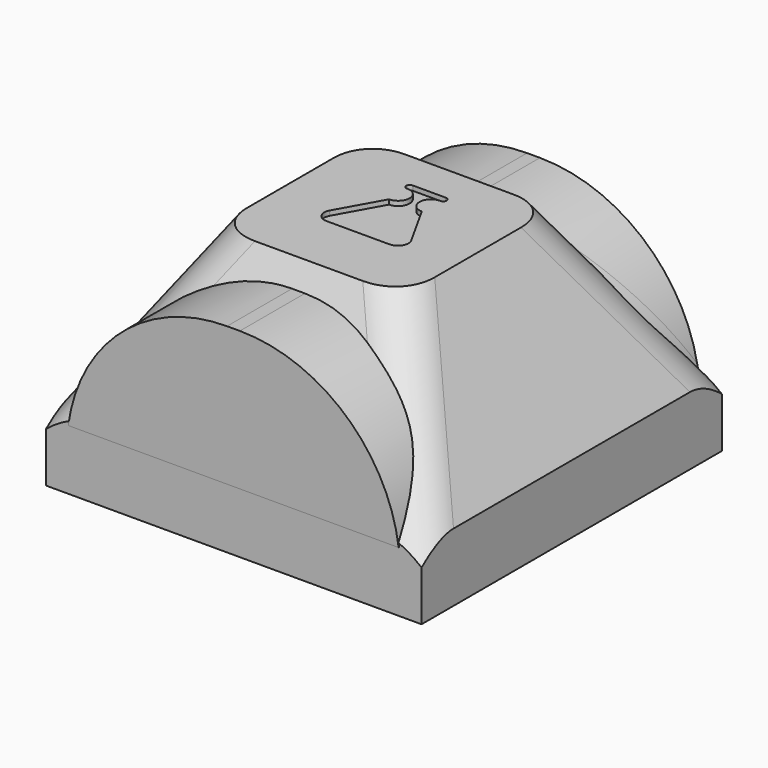
from build123d import *

# Parameters (mm, degrees)
F0_W          = 40.64
F0_H          = 40.64
F1_DEPTH      = 23.876
F2_SIZE2      = 10.16
F2_SIZE       = 16.51
F4_DEPTH      = 5.5372
F4_DEPTH_BACK = 35.052
F6_DEPTH      = 0.508
F7_T4_DEPTH   = 41.0469310155
F7_S5_R       = 17.3367265746
F7_T6_DEPTH   = 25
F7_T10_DEPTH  = 41.0469310155
F7_S11_R      = 17.3367265746
F7_T12_DEPTH  = 25
F7_T16_DEPTH  = 41.0469310155
F7_S17_R      = 17.3367265746
F7_T18_DEPTH  = 25
F7_T23_DEPTH  = 41.0469310155
F7_S24_R      = 17.3367265746
F7_T25_DEPTH  = 25
F7_T30_DEPTH  = 41.0469310155
F7_S31_R      = 17.3367265746
F7_T32_DEPTH  = 25
F7_T37_DEPTH  = 41.0469310155
F7_S39_R      = 17.3367265746
F7_T40_DEPTH  = 25
F7_T44_DEPTH  = 41.0469310155
F7_S46_R      = 17.3367265746
F7_T47_DEPTH  = 25
F7_T51_DEPTH  = 41.0469310155
F7_S53_R      = 17.3367265746
F7_T54_DEPTH  = 25


# Not quite as in the source:
# - a fillet or chamfer that OpenCascade refuses, or shapes differently, is made with other operations: its cross-section is extruded or revolved along the edge and cut away or added


with BuildPart() as f1:
    # F0 (on Top) → F1 (new body)
    with BuildSketch(Plane.XY):
        with Locations((-20.32, 14.8309261845)):
            Rectangle(F0_W, F0_H)
    extrude(amount=F1_DEPTH)

    # F2
    f2_edges = [f1.edges().sort_by_distance(p)[0] for p in [
        (0, 14.830926, 23.876),
        (-20.32, 35.150926, 23.876),
        (-40.64, 14.830926, 23.876),
        (-20.32, -5.489074, 23.876),
    ]]
    chamfer(f2_edges, length=F2_SIZE, length2=F2_SIZE2)

    # F3 (on Front) → F4 (join, two sides)
    with BuildSketch(Plane.XZ) as f4_sk:
        with BuildLine():
            Line((-19.622727835, 21.5899987397), (-21.017272165, 21.5899987397))
            ThreePointArc((-21.017272165, 21.5899987397), (-32.4394065874, 17.2953936781), (-38.2026230943, 6.5392734254))
            Line((-38.2026230943, 6.5392734254), (-2.4373769057, 6.5392734254))
            ThreePointArc((-2.4373769057, 6.5392734254), (-8.2005934126, 17.2953936781), (-19.622727835, 21.5899987397))
        make_face()
    extrude(amount=F4_DEPTH)
    extrude(f4_sk.sketch, amount=-F4_DEPTH_BACK)

    # F5 (on face) → F6 (cut)
    with BuildSketch(Plane.XY.offset(23.876)):
        with BuildLine():
            Line((-20.32, 11.3146617191), (-20.32, 20.958676386))
            Line((-20.32, 20.958676386), (-22.098, 20.958676386))
            ThreePointArc((-22.098, 20.958676386), (-22.5080143202, 20.5929218839), (-22.1218966733, 20.2020238648))
            ThreePointArc((-22.1218966733, 20.2020238648), (-20.8577108363, 18.9738562556), (-22.098, 17.7215606446))
            Line((-22.098, 17.7215606446), (-24.7307707736, 12.9957624854))
            ThreePointArc((-24.7307707736, 12.9957624854), (-24.7178678661, 11.8725673854), (-23.7429447999, 11.3146617191))
            Line((-23.7429447999, 11.3146617191), (-20.32, 11.3146617191))
        make_face()
        with BuildLine():
            Line((-18.542, 20.958676386), (-20.32, 20.958676386))
            Line((-20.32, 20.958676386), (-20.32, 11.3146617191))
            Line((-20.32, 11.3146617191), (-16.8970552001, 11.3146617191))
            ThreePointArc((-16.8970552001, 11.3146617191), (-15.9221321339, 11.8725673854), (-15.9092292264, 12.9957624854))
            Line((-15.9092292264, 12.9957624854), (-18.542, 17.7215606446))
            ThreePointArc((-18.542, 17.7215606446), (-19.7822891637, 18.9738562556), (-18.5181033267, 20.2020238648))
            ThreePointArc((-18.5181033267, 20.2020238648), (-18.1319856798, 20.5929218839), (-18.542, 20.958676386))
        make_face()
    extrude(amount=-F6_DEPTH, mode=Mode.SUBTRACT)

    # F7: fillet of radius 5.08 on 4 edges, made by hand


with BuildPart() as f7_tool2:
    # F7_s3 → F7_t4 (new body)
    with BuildSketch(Plane(origin=(-11.8080697784, -11.8080697784, -19.18811339), x_dir=(-0.7071067812, 0.7071067812, 0), z_dir=(0.4642070825, 0.4642070825, 0.7543365091))):
        with BuildLine():
            ThreePointArc((21.7962143454, 27.1330755892), (24.85545827, 28.157532887), (27.9147021947, 27.1330755892))
            Line((27.9147021947, 27.1330755892), (24.85545827, 29.4407749719))
            Line((24.85545827, 29.4407749719), (21.7962143454, 27.1330755892))
        make_face()
    extrude(amount=F7_T4_DEPTH)

    # F7_s5 → F7_t6 (cut, symmetric)
    with BuildSketch(Plane.XZ.offset(-0.8)):
        with Locations((-21.017272165, 4.253272165)):
            Circle(F7_S5_R)
    extrude(amount=F7_T6_DEPTH, both=True, mode=Mode.SUBTRACT)


with BuildPart() as f1_1:
    add(f1.part)

    # F7_t1: cut F7_tool2
    add(f7_tool2.part, mode=Mode.SUBTRACT)


with BuildPart() as f7_tool8:
    # F7_s9 → F7_t10 (new body)
    with BuildSketch(Plane(origin=(3.050628701, -3.050628701, -4.9572716391), x_dir=(-0.7071067812, -0.7071067812, 0), z_dir=(-0.4642070825, 0.4642070825, 0.7543365091))):
        with BuildLine():
            ThreePointArc((0.8221173927, 5.4558434178), (3.8813613174, 6.4803007156), (6.9406052421, 5.4558434178))
            Line((6.9406052421, 5.4558434178), (3.8813613174, 7.7635428005))
            Line((3.8813613174, 7.7635428005), (0.8221173927, 5.4558434178))
        make_face()
    extrude(amount=F7_T10_DEPTH)

    # F7_s11 → F7_t12 (cut, symmetric)
    with BuildSketch(Plane.XZ.offset(-0.8)):
        with Locations((-19.622727835, 4.253272165)):
            Circle(F7_S11_R)
    extrude(amount=F7_T12_DEPTH, both=True, mode=Mode.SUBTRACT)


with BuildPart() as f1_2:
    add(f1_1.part)

    # F7_t7: cut F7_tool8
    add(f7_tool8.part, mode=Mode.SUBTRACT)


with BuildPart() as f7_tool14:
    # F7_s15 → F7_t16 (new body)
    with BuildSketch(Plane(origin=(9.442408336, 9.442408336, -15.3439135461), x_dir=(0.7071067812, -0.7071067812, 0), z_dir=(-0.4642070825, -0.4642070825, 0.7543365091))):
        with BuildLine():
            ThreePointArc((-21.7962143454, 21.2773704954), (-24.85545827, 22.3018277932), (-27.9147021947, 21.2773704954))
            Line((-27.9147021947, 21.2773704954), (-24.85545827, 23.5850698781))
            Line((-24.85545827, 23.5850698781), (-21.7962143454, 21.2773704954))
        make_face()
    extrude(amount=F7_T16_DEPTH)

    # F7_s17 → F7_t18 (cut, symmetric)
    with BuildSketch(Plane.XZ.offset(-28.8)):
        with Locations((-19.622727835, 4.253272165)):
            Circle(F7_S17_R)
    extrude(amount=F7_T18_DEPTH, both=True, mode=Mode.SUBTRACT)

    split(bisect_by=Plane.XZ.offset(-35.052), keep=Keep.BOTTOM)


with BuildPart() as f1_3:
    add(f1_2.part)

    # F7_t13: cut F7_tool14
    add(f7_tool14.part, mode=Mode.SUBTRACT)


with BuildPart() as f7_tool21:
    # F7_s22 → F7_t23 (new body)
    with BuildSketch(Plane(origin=(9.442408336, 9.442408336, -15.3439135461), x_dir=(0.7071067812, -0.7071067812, 0), z_dir=(-0.4642070825, -0.4642070825, 0.7543365091))):
        with BuildLine():
            ThreePointArc((-21.7962143454, 21.2773704954), (-24.85545827, 22.3018277932), (-27.9147021947, 21.2773704954))
            Line((-27.9147021947, 21.2773704954), (-24.85545827, 23.5850698781))
            Line((-24.85545827, 23.5850698781), (-21.7962143454, 21.2773704954))
        make_face()
    extrude(amount=F7_T23_DEPTH)

    # F7_s24 → F7_t25 (intersect, symmetric)
    with BuildSketch(Plane.XZ.offset(-28.8)):
        with Locations((-19.622727835, 4.253272165)):
            Circle(F7_S24_R)
    extrude(amount=F7_T25_DEPTH, both=True, mode=Mode.INTERSECT)

    split(bisect_by=Plane.XZ.offset(-35.052), keep=Keep.BOTTOM)


with BuildPart() as f1_4:
    add(f1_3.part)

    # F7_t20: cut F7_tool21
    add(f7_tool21.part, mode=Mode.SUBTRACT)


with BuildPart() as f7_tool28:
    # F7_s29 → F7_t30 (new body)
    with BuildSketch(Plane(origin=(9.442408336, 9.442408336, -15.3439135461), x_dir=(0.7071067812, -0.7071067812, 0), z_dir=(-0.4642070825, -0.4642070825, 0.7543365091))):
        with BuildLine():
            ThreePointArc((-21.7962143454, 21.2773704954), (-24.85545827, 22.3018277932), (-27.9147021947, 21.2773704954))
            Line((-27.9147021947, 21.2773704954), (-24.85545827, 23.5850698781))
            Line((-24.85545827, 23.5850698781), (-21.7962143454, 21.2773704954))
        make_face()
    extrude(amount=F7_T30_DEPTH)

    # F7_s31 → F7_t32 (cut, symmetric)
    with BuildSketch(Plane.XZ.offset(-28.8)):
        with Locations((-19.622727835, 4.253272165)):
            Circle(F7_S31_R)
    extrude(amount=F7_T32_DEPTH, both=True, mode=Mode.SUBTRACT)

    split(bisect_by=Plane.XZ.offset(-35.052), keep=Keep.TOP)


with BuildPart() as f1_5:
    add(f1_4.part)

    # F7_t27: cut F7_tool28
    add(f7_tool28.part, mode=Mode.SUBTRACT)


with BuildPart() as f7_tool35:
    # F7_s36 → F7_t37 (new body)
    with BuildSketch(Plane(origin=(-18.1998494135, 18.1998494135, -29.5747552969), x_dir=(0.7071067812, 0.7071067812, 0), z_dir=(0.4642070825, -0.4642070825, 0.7543365091))):
        with BuildLine():
            ThreePointArc((-0.8221173927, 42.9546026668), (-3.8813613174, 43.9790599646), (-6.9406052421, 42.9546026668))
            Line((-6.9406052421, 42.9546026668), (-3.8813613174, 45.2623020495))
            Line((-3.8813613174, 45.2623020495), (-0.8221173927, 42.9546026668))
        make_face()
    extrude(amount=F7_T37_DEPTH)

    split(bisect_by=Plane.XZ.offset(-35.052), keep=Keep.BOTTOM)

    # F7_s39 → F7_t40 (cut, symmetric)
    with BuildSketch(Plane.XZ.offset(-28.8)):
        with Locations((-21.017272165, 4.253272165)):
            Circle(F7_S39_R)
    extrude(amount=F7_T40_DEPTH, both=True, mode=Mode.SUBTRACT)


with BuildPart() as f1_6:
    add(f1_5.part)

    # F7_t34: cut F7_tool35
    add(f7_tool35.part, mode=Mode.SUBTRACT)


with BuildPart() as f7_tool42:
    # F7_s43 → F7_t44 (new body)
    with BuildSketch(Plane(origin=(-18.1998494135, 18.1998494135, -29.5747552969), x_dir=(0.7071067812, 0.7071067812, 0), z_dir=(0.4642070825, -0.4642070825, 0.7543365091))):
        with BuildLine():
            ThreePointArc((-0.8221173927, 42.9546026668), (-3.8813613174, 43.9790599646), (-6.9406052421, 42.9546026668))
            Line((-6.9406052421, 42.9546026668), (-3.8813613174, 45.2623020495))
            Line((-3.8813613174, 45.2623020495), (-0.8221173927, 42.9546026668))
        make_face()
    extrude(amount=F7_T44_DEPTH)

    split(bisect_by=Plane.XZ.offset(-35.052), keep=Keep.TOP)

    # F7_s46 → F7_t47 (cut, symmetric)
    with BuildSketch(Plane.XZ.offset(-28.8)):
        with Locations((-21.017272165, 4.253272165)):
            Circle(F7_S46_R)
    extrude(amount=F7_T47_DEPTH, both=True, mode=Mode.SUBTRACT)


with BuildPart() as f1_7:
    add(f1_6.part)

    # F7_t41: cut F7_tool42
    add(f7_tool42.part, mode=Mode.SUBTRACT)


with BuildPart() as f7_tool49:
    # F7_s50 → F7_t51 (new body)
    with BuildSketch(Plane(origin=(-18.1998494135, 18.1998494135, -29.5747552969), x_dir=(0.7071067812, 0.7071067812, 0), z_dir=(0.4642070825, -0.4642070825, 0.7543365091))):
        with BuildLine():
            ThreePointArc((-0.8221173927, 42.9546026668), (-3.8813613174, 43.9790599646), (-6.9406052421, 42.9546026668))
            Line((-6.9406052421, 42.9546026668), (-3.8813613174, 45.2623020495))
            Line((-3.8813613174, 45.2623020495), (-0.8221173927, 42.9546026668))
        make_face()
    extrude(amount=F7_T51_DEPTH)

    split(bisect_by=Plane.XZ.offset(-35.052), keep=Keep.BOTTOM)

    # F7_s53 → F7_t54 (intersect, symmetric)
    with BuildSketch(Plane.XZ.offset(-28.8)):
        with Locations((-21.017272165, 4.253272165)):
            Circle(F7_S53_R)
    extrude(amount=F7_T54_DEPTH, both=True, mode=Mode.INTERSECT)


with BuildPart() as f1_8:
    add(f1_7.part)

    # F7_t48: cut F7_tool49
    add(f7_tool49.part, mode=Mode.SUBTRACT)


solid = f1_8.part
